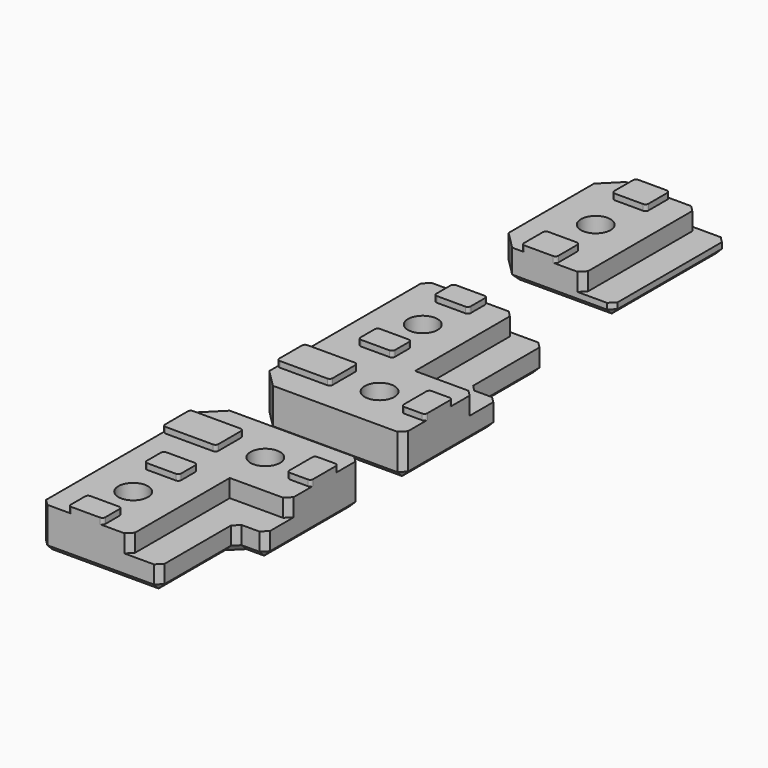
from build123d import *

# Parameters (mm, degrees)
F0_W      = 9
F0_H      = 5.8
F0_W_2    = 4
F0_W_3    = 5.8
F0_H_2    = 4
F1_DEPTH  = 4
F0_R      = 2.5
F2_DEPTH  = 3
F0_R_2    = 5.5
F0_H_3    = 5
F3_DEPTH  = 4
F4_DEPTH  = 4
F0_W_4    = 5
F0_H_4    = 24
F5_DEPTH  = 2
F6_SIZE   = 3
F6_2_SIZE = 3
F7_SIZE   = 1
F7_2_SIZE = 1
F8_DEPTH  = 0.2
F9_R      = 0.5
F9_2_R    = 0.5


with BuildPart() as f1:
    # F0 (on Top) → F1 (new body)
    with BuildSketch(Plane.XY):
        with BuildLine():
            Line((-211.1212035418, 81.4429656104), (-211.1212035418, 55.8429656104))
            Line((-211.1212035418, 55.8429656104), (-202.1212035418, 55.8429656104))
            Line((-202.1212035418, 55.8429656104), (-200.79453212, 55.8429656104))
            ThreePointArc((-200.79453212, 55.8429656104), (-196.1212035418, 58.4429656104), (-191.4478749635, 55.8429656104))
            Line((-191.4478749635, 55.8429656104), (-190.1212035418, 55.8429656104))
            Line((-190.1212035418, 55.8429656104), (-186.1212035418, 55.8429656104))
            Line((-186.1212035418, 55.8429656104), (-186.1212035418, 60.4429656104))
            Line((-186.1212035418, 60.4429656104), (-196.1212035418, 60.4429656104))
            Line((-196.1212035418, 60.4429656104), (-196.1212035418, 81.4429656104))
            Line((-196.1212035418, 81.4429656104), (-200.7212035418, 81.4429656104))
            Line((-200.7212035418, 81.4429656104), (-200.7212035418, 77.4429656104))
            Line((-200.7212035418, 77.4429656104), (-200.7212035418, 76.1162941886))
            ThreePointArc((-200.7212035418, 76.1162941886), (-198.8149576055, 74.1169140018), (-198.1212035418, 71.4429656104))
            ThreePointArc((-198.1212035418, 71.4429656104), (-198.8149576055, 68.769017219), (-200.7212035418, 66.7696370322))
            Line((-200.7212035418, 66.7696370322), (-200.7212035418, 65.4429656104))
            Line((-200.7212035418, 65.4429656104), (-200.7212035418, 61.4429656104))
            Line((-200.7212035418, 61.4429656104), (-206.5212035418, 61.4429656104))
            Line((-206.5212035418, 61.4429656104), (-206.5212035418, 65.4429656104))
            Line((-206.5212035418, 65.4429656104), (-206.5212035418, 66.7696370322))
            ThreePointArc((-206.5212035418, 66.7696370322), (-209.1212035418, 71.4429656104), (-206.5212035418, 76.1162941886))
            Line((-206.5212035418, 76.1162941886), (-206.5212035418, 77.4429656104))
            Line((-206.5212035418, 77.4429656104), (-206.5212035418, 81.4429656104))
            Line((-206.5212035418, 81.4429656104), (-211.1212035418, 81.4429656104))
        make_face()
        with BuildLine():
            Line((-202.1212035418, 55.8429656104), (-202.1212035418, 50.0429656104))
            Line((-202.1212035418, 50.0429656104), (-200.79453212, 50.0429656104))
            ThreePointArc((-200.79453212, 50.0429656104), (-201.6212035418, 52.9429656104), (-200.79453212, 55.8429656104))
            Line((-200.79453212, 55.8429656104), (-202.1212035418, 55.8429656104))
        make_face()
        with Locations((-206.6212035418, 52.9429656104)):
            Rectangle(F0_W, F0_H)
        with BuildLine():
            Line((-211.1212035418, 50.0429656104), (-211.1212035418, 45.4429656104))
            Line((-211.1212035418, 45.4429656104), (-186.1212035418, 45.4429656104))
            Line((-186.1212035418, 45.4429656104), (-186.1212035418, 50.0429656104))
            Line((-186.1212035418, 50.0429656104), (-190.1212035418, 50.0429656104))
            Line((-190.1212035418, 50.0429656104), (-191.4478749635, 50.0429656104))
            ThreePointArc((-191.4478749635, 50.0429656104), (-196.1212035418, 47.4429656104), (-200.79453212, 50.0429656104))
            Line((-200.79453212, 50.0429656104), (-202.1212035418, 50.0429656104))
            Line((-202.1212035418, 50.0429656104), (-211.1212035418, 50.0429656104))
        make_face()
        with BuildLine():
            Line((-191.4478749635, 50.0429656104), (-190.1212035418, 50.0429656104))
            Line((-190.1212035418, 50.0429656104), (-190.1212035418, 55.8429656104))
            Line((-190.1212035418, 55.8429656104), (-191.4478749635, 55.8429656104))
            ThreePointArc((-191.4478749635, 55.8429656104), (-190.831907408, 54.4507276639), (-190.6212035418, 52.9429656104))
            ThreePointArc((-190.6212035418, 52.9429656104), (-190.831907408, 51.4352035569), (-191.4478749635, 50.0429656104))
        make_face()
        with Locations((-188.1212035418, 52.9429656104)):
            Rectangle(F0_W_2, F0_H)
        with Locations((-203.6212035418, 63.4429656104)):
            Rectangle(F0_W_3, F0_H_2)
        with BuildLine():
            ThreePointArc((-200.7212035418, 66.7696370322), (-203.6212035418, 65.9429656104), (-206.5212035418, 66.7696370322))
            Line((-206.5212035418, 66.7696370322), (-206.5212035418, 65.4429656104))
            Line((-206.5212035418, 65.4429656104), (-200.7212035418, 65.4429656104))
            Line((-200.7212035418, 65.4429656104), (-200.7212035418, 66.7696370322))
        make_face()
        with BuildLine():
            Line((-200.7212035418, 77.4429656104), (-206.5212035418, 77.4429656104))
            Line((-206.5212035418, 77.4429656104), (-206.5212035418, 76.1162941886))
            ThreePointArc((-206.5212035418, 76.1162941886), (-203.6212035418, 76.9429656104), (-200.7212035418, 76.1162941886))
            Line((-200.7212035418, 76.1162941886), (-200.7212035418, 77.4429656104))
        make_face()
        with Locations((-203.6212035418, 79.4429656104)):
            Rectangle(F0_W_3, F0_H_2)
    extrude(amount=-F1_DEPTH)

    # F0 (on Top) → F2 (join)
    with BuildSketch(Plane.XY):
        with BuildLine():
            Line((-211.1212035418, 81.4429656104), (-211.1212035418, 55.8429656104))
            Line((-211.1212035418, 55.8429656104), (-202.1212035418, 55.8429656104))
            Line((-202.1212035418, 55.8429656104), (-200.79453212, 55.8429656104))
            ThreePointArc((-200.79453212, 55.8429656104), (-196.1212035418, 58.4429656104), (-191.4478749635, 55.8429656104))
            Line((-191.4478749635, 55.8429656104), (-190.1212035418, 55.8429656104))
            Line((-190.1212035418, 55.8429656104), (-186.1212035418, 55.8429656104))
            Line((-186.1212035418, 55.8429656104), (-186.1212035418, 60.4429656104))
            Line((-186.1212035418, 60.4429656104), (-196.1212035418, 60.4429656104))
            Line((-196.1212035418, 60.4429656104), (-196.1212035418, 81.4429656104))
            Line((-196.1212035418, 81.4429656104), (-200.7212035418, 81.4429656104))
            Line((-200.7212035418, 81.4429656104), (-200.7212035418, 77.4429656104))
            Line((-200.7212035418, 77.4429656104), (-200.7212035418, 76.1162941886))
            ThreePointArc((-200.7212035418, 76.1162941886), (-198.8149576055, 74.1169140018), (-198.1212035418, 71.4429656104))
            ThreePointArc((-198.1212035418, 71.4429656104), (-198.8149576055, 68.769017219), (-200.7212035418, 66.7696370322))
            Line((-200.7212035418, 66.7696370322), (-200.7212035418, 65.4429656104))
            Line((-200.7212035418, 65.4429656104), (-200.7212035418, 61.4429656104))
            Line((-200.7212035418, 61.4429656104), (-206.5212035418, 61.4429656104))
            Line((-206.5212035418, 61.4429656104), (-206.5212035418, 65.4429656104))
            Line((-206.5212035418, 65.4429656104), (-206.5212035418, 66.7696370322))
            ThreePointArc((-206.5212035418, 66.7696370322), (-209.1212035418, 71.4429656104), (-206.5212035418, 76.1162941886))
            Line((-206.5212035418, 76.1162941886), (-206.5212035418, 77.4429656104))
            Line((-206.5212035418, 77.4429656104), (-206.5212035418, 81.4429656104))
            Line((-206.5212035418, 81.4429656104), (-211.1212035418, 81.4429656104))
        make_face()
        with Locations((-203.6212035418, 63.4429656104)):
            Rectangle(F0_W_3, F0_H_2)
        with BuildLine():
            ThreePointArc((-200.7212035418, 66.7696370322), (-203.6212035418, 65.9429656104), (-206.5212035418, 66.7696370322))
            Line((-206.5212035418, 66.7696370322), (-206.5212035418, 65.4429656104))
            Line((-206.5212035418, 65.4429656104), (-200.7212035418, 65.4429656104))
            Line((-200.7212035418, 65.4429656104), (-200.7212035418, 66.7696370322))
        make_face()
        with BuildLine():
            Line((-202.1212035418, 55.8429656104), (-202.1212035418, 50.0429656104))
            Line((-202.1212035418, 50.0429656104), (-200.79453212, 50.0429656104))
            ThreePointArc((-200.79453212, 50.0429656104), (-201.6212035418, 52.9429656104), (-200.79453212, 55.8429656104))
            Line((-200.79453212, 55.8429656104), (-202.1212035418, 55.8429656104))
        make_face()
        with Locations((-206.6212035418, 52.9429656104)):
            Rectangle(F0_W, F0_H)
        with BuildLine():
            Line((-211.1212035418, 50.0429656104), (-211.1212035418, 45.4429656104))
            Line((-211.1212035418, 45.4429656104), (-186.1212035418, 45.4429656104))
            Line((-186.1212035418, 45.4429656104), (-186.1212035418, 50.0429656104))
            Line((-186.1212035418, 50.0429656104), (-190.1212035418, 50.0429656104))
            Line((-190.1212035418, 50.0429656104), (-191.4478749635, 50.0429656104))
            ThreePointArc((-191.4478749635, 50.0429656104), (-196.1212035418, 47.4429656104), (-200.79453212, 50.0429656104))
            Line((-200.79453212, 50.0429656104), (-202.1212035418, 50.0429656104))
            Line((-202.1212035418, 50.0429656104), (-211.1212035418, 50.0429656104))
        make_face()
        with BuildLine():
            Line((-191.4478749635, 50.0429656104), (-190.1212035418, 50.0429656104))
            Line((-190.1212035418, 50.0429656104), (-190.1212035418, 55.8429656104))
            Line((-190.1212035418, 55.8429656104), (-191.4478749635, 55.8429656104))
            ThreePointArc((-191.4478749635, 55.8429656104), (-190.831907408, 54.4507276639), (-190.6212035418, 52.9429656104))
            ThreePointArc((-190.6212035418, 52.9429656104), (-190.831907408, 51.4352035569), (-191.4478749635, 50.0429656104))
        make_face()
        with Locations((-188.1212035418, 52.9429656104)):
            Rectangle(F0_W_2, F0_H)
        with BuildLine():
            ThreePointArc((-200.7212035418, 76.1162941886), (-203.6212035418, 76.9429656104), (-206.5212035418, 76.1162941886))
            ThreePointArc((-206.5212035418, 76.1162941886), (-209.1212035418, 71.4429656104), (-206.5212035418, 66.7696370322))
            ThreePointArc((-206.5212035418, 66.7696370322), (-203.6212035418, 65.9429656104), (-200.7212035418, 66.7696370322))
            ThreePointArc((-200.7212035418, 66.7696370322), (-198.8149576055, 68.769017219), (-198.1212035418, 71.4429656104))
            ThreePointArc((-198.1212035418, 71.4429656104), (-198.8149576055, 74.1169140018), (-200.7212035418, 76.1162941886))
        make_face()
        with Locations((-203.6212035418, 71.4429656104)):
            Circle(F0_R, mode=Mode.SUBTRACT)
        with BuildLine():
            Line((-200.7212035418, 77.4429656104), (-206.5212035418, 77.4429656104))
            Line((-206.5212035418, 77.4429656104), (-206.5212035418, 76.1162941886))
            ThreePointArc((-206.5212035418, 76.1162941886), (-203.6212035418, 76.9429656104), (-200.7212035418, 76.1162941886))
            Line((-200.7212035418, 76.1162941886), (-200.7212035418, 77.4429656104))
        make_face()
        with Locations((-203.6212035418, 79.4429656104)):
            Rectangle(F0_W_3, F0_H_2)
        with BuildLine():
            ThreePointArc((-200.79453212, 55.8429656104), (-201.6212035418, 52.9429656104), (-200.79453212, 50.0429656104))
            ThreePointArc((-200.79453212, 50.0429656104), (-196.1212035418, 47.4429656104), (-191.4478749635, 50.0429656104))
            ThreePointArc((-191.4478749635, 50.0429656104), (-190.831907408, 51.4352035569), (-190.6212035418, 52.9429656104))
            ThreePointArc((-190.6212035418, 52.9429656104), (-190.831907408, 54.4507276639), (-191.4478749635, 55.8429656104))
            ThreePointArc((-191.4478749635, 55.8429656104), (-196.1212035418, 58.4429656104), (-200.79453212, 55.8429656104))
        make_face()
        with Locations((-196.1212035418, 52.9429656104)):
            Circle(F0_R, mode=Mode.SUBTRACT)
    extrude(amount=F2_DEPTH)

    # F0 (on Top) → F3 (join)
    with BuildSketch(Plane.XY):
        with Locations((-203.6212035418, 63.4429656104)):
            Rectangle(F0_W_3, F0_H_2)
        with Locations((-203.6212035418, 79.4429656104)):
            Rectangle(F0_W_3, F0_H_2)
        with Locations((-206.6212035418, 52.9429656104)):
            Rectangle(F0_W, F0_H)
        with Locations((-188.1212035418, 52.9429656104)):
            Rectangle(F0_W_2, F0_H)
    extrude(amount=F3_DEPTH)

    # F0 (on Top) → F4 (join)
    with BuildSketch(Plane.XY):
        Polygon((-196.1212035418, 60.4429656104), (-186.1212035418, 60.4429656104), (-186.1212035418, 65.4429656104), (-191.1212035418, 65.4429656104), (-191.1212035418, 81.4429656104), (-196.1212035418, 81.4429656104), align=None)
    extrude(amount=-F4_DEPTH)

    # F6
    f6_edges = [f1.edges().sort_by_distance(p)[0] for p in [
        (-211.121204, 45.442966, -0.5),
    ]]
    chamfer(f6_edges, length=F6_SIZE)

    # F7
    f7_edges = [f1.edges().sort_by_distance(p)[0] for p in [
        (-186.121204, 45.442966, -0.5),
        (-196.121204, 81.442966, 1.5),
        (-197.121204, 45.442966, -4),
        (-209.621204, 46.942966, -4),
        (-211.121204, 64.942966, -4),
        (-186.121204, 60.442966, 1.5),
        (-211.121204, 81.442966, -0.5),
        (-191.121204, 65.442966, -2),
        (-191.121204, 73.442966, -4),
        (-188.621204, 65.442966, -4),
        (-201.121204, 81.442966, -4),
        (-186.121204, 55.442966, -4),
        (-191.121204, 81.442966, -2),
        (-186.121204, 65.442966, -2),
    ]]
    chamfer(f7_edges, length=F7_SIZE)

    # F0 (on Top) → F8 (join)
    with BuildSketch(Plane.XY):
        with Locations((-203.6212035418, 71.4429656104)):
            Circle(F0_R)
        with Locations((-196.1212035418, 52.9429656104)):
            Circle(F0_R)
    extrude(amount=F8_DEPTH)

    # F9
    f9_edges = [f1.edges().sort_by_distance(p)[0] for p in [
        (-186.121204, 55.842966, 3.5),
        (-190.121204, 55.842966, 3.5),
        (-186.121204, 50.042966, 3.5),
        (-190.121204, 50.042966, 3.5),
        (-200.721204, 61.442966, 3.5),
        (-206.521204, 61.442966, 3.5),
        (-206.521204, 65.442966, 3.5),
        (-200.721204, 65.442966, 3.5),
        (-200.721204, 81.442966, 3.5),
        (-206.521204, 81.442966, 3.5),
        (-206.521204, 77.442966, 3.5),
        (-200.721204, 77.442966, 3.5),
        (-202.121204, 50.042966, 3.5),
        (-202.121204, 55.842966, 3.5),
        (-211.121204, 50.042966, 3.5),
        (-211.121204, 55.842966, 3.5),
    ]]
    fillet(f9_edges, radius=F9_R)


with BuildPart() as f2:
    # F0 (on Top) → F2, piece 2 (new body)
    with BuildSketch(Plane.XY):
        Polygon((-211.1212035418, 119.9315821528), (-211.1212035418, 95.9315821528), (-206.5212035418, 95.9315821528), (-206.5212035418, 100.9315821528), (-200.7212035418, 100.9315821528), (-200.7212035418, 95.9315821528), (-196.1212035418, 95.9315821528), (-196.1212035418, 119.9315821528), (-200.7212035418, 119.9315821528), (-200.7212035418, 114.9315821528), (-206.5212035418, 114.9315821528), (-206.5212035418, 119.9315821528), align=None)
        with Locations((-203.6212035418, 107.9315821528)):
            Circle(F0_R_2, mode=Mode.SUBTRACT)
        with Locations((-203.6212035418, 98.4315821528)):
            Rectangle(F0_W_3, F0_H_3)
        with Locations((-203.6212035418, 117.4315821528)):
            Rectangle(F0_W_3, F0_H_3)
        with Locations((-203.6212035418, 107.9315821528)):
            Circle(F0_R_2)
        with Locations((-203.6212035418, 107.9315821528)):
            Circle(F0_R, mode=Mode.SUBTRACT)
    extrude(amount=F2_DEPTH)

    # F0 (on Top) → F3, piece 2 (join)
    with BuildSketch(Plane.XY):
        with Locations((-203.6212035418, 98.4315821528)):
            Rectangle(F0_W_3, F0_H_3)
        with Locations((-203.6212035418, 117.4315821528)):
            Rectangle(F0_W_3, F0_H_3)
    extrude(amount=F3_DEPTH)

    # F0 (on Top) → F5 (join)
    with BuildSketch(Plane.XY):
        Polygon((-211.1212035418, 119.9315821528), (-211.1212035418, 95.9315821528), (-206.5212035418, 95.9315821528), (-206.5212035418, 100.9315821528), (-200.7212035418, 100.9315821528), (-200.7212035418, 95.9315821528), (-196.1212035418, 95.9315821528), (-196.1212035418, 119.9315821528), (-200.7212035418, 119.9315821528), (-200.7212035418, 114.9315821528), (-206.5212035418, 114.9315821528), (-206.5212035418, 119.9315821528), align=None)
        with Locations((-203.6212035418, 107.9315821528)):
            Circle(F0_R_2, mode=Mode.SUBTRACT)
        with Locations((-193.6212035418, 107.9315821528)):
            Rectangle(F0_W_4, F0_H_4)
        with Locations((-203.6212035418, 98.4315821528)):
            Rectangle(F0_W_3, F0_H_3)
        with Locations((-203.6212035418, 117.4315821528)):
            Rectangle(F0_W_3, F0_H_3)
    extrude(amount=-F5_DEPTH)

    # F6#2
    f6_2_edges = [f2.edges().sort_by_distance(p)[0] for p in [
        (-211.121204, 95.931582, 0.5),
        (-211.121204, 119.931582, 0.5),
    ]]
    chamfer(f6_2_edges, length=F6_2_SIZE)

    # F7#2
    f7_2_edges = [f2.edges().sort_by_distance(p)[0] for p in [
        (-196.121204, 95.931582, 1.5),
        (-196.121204, 119.931582, 1.5),
        (-191.121204, 119.931582, -1),
        (-191.121204, 95.931582, -1),
        (-191.121204, 107.931582, -2),
        (-199.621204, 119.931582, -2),
        (-211.121204, 107.931582, -2),
        (-209.621204, 118.431582, -2),
        (-209.621204, 97.431582, -2),
        (-199.621204, 95.931582, -2),
    ]]
    chamfer(f7_2_edges, length=F7_2_SIZE)

    # F0 (on Top) → F8, piece 2 (join)
    with BuildSketch(Plane.XY):
        with Locations((-203.6212035418, 107.9315821528)):
            Circle(F0_R)
    extrude(amount=F8_DEPTH)

    # F9#2
    f9_2_edges = [f2.edges().sort_by_distance(p)[0] for p in [
        (-206.521204, 95.931582, 3.5),
        (-206.521204, 100.931582, 3.5),
        (-200.721204, 95.931582, 3.5),
        (-200.721204, 100.931582, 3.5),
        (-200.721204, 114.931582, 3.5),
        (-206.521204, 114.931582, 3.5),
        (-206.521204, 119.931582, 3.5),
        (-200.721204, 119.931582, 3.5),
    ]]
    fillet(f9_2_edges, radius=F9_2_R)


with BuildPart() as f10_1:
    # F10: instance of F1
    add(f1.part.mirror(Plane(origin=(-197.6212035418, 45.4429656104, 0), x_dir=(1, 0, 0), z_dir=(0, -1, 0))))


with BuildPart() as f10_1_1:
    # F11: moved
    add(f10_1.part.moved(Location((0, -9.1, 0))))


solid = Compound([f1.part, f2.part, f10_1_1.part])
